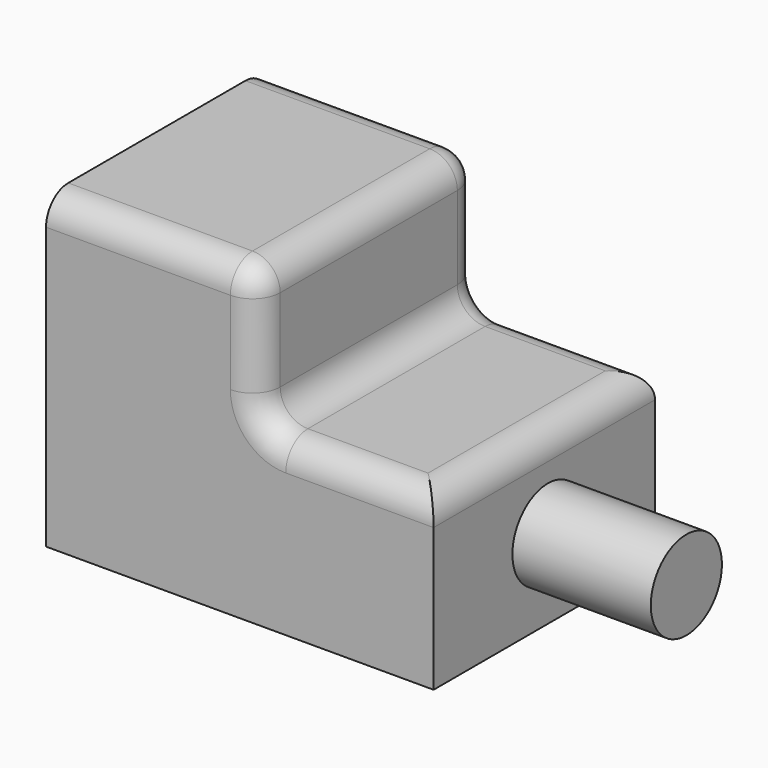
from build123d import *

# Parameters (mm, degrees)
F0_W     = 70
F0_H     = 50
F1_DEPTH = 55.8
F2_R     = 5
F3_R     = 5
F4_W     = 31.709628962
F4_H     = 40
F5_DEPTH = 25
F6_R     = 5
F7_R     = 8.0311344771
F8_DEPTH = 25


with BuildPart() as f1:
    # F0 (on Top) → F1 (new body)
    with BuildSketch(Plane.XY):
        with Locations((-9.0379202738, -0.8199248582)):
            Rectangle(F0_W, F0_H)
    extrude(amount=F1_DEPTH)

    # F2
    f2_edges = [f1.edges().sort_by_distance(p)[0] for p in [
        (-9.03792, -25.819925, 55.8),
    ]]
    fillet(f2_edges, radius=F2_R)

    # F3
    f3_edges = [f1.edges().sort_by_distance(p)[0] for p in [
        (-9.03792, 24.180075, 55.8),
    ]]
    fillet(f3_edges, radius=F3_R)

    # F4 (on face) → F5 (cut)
    with BuildSketch(Plane.XY.offset(55.8)):
        Polygon((30.625000596, 31.9975502789), (-5.7475492358, 31.9975502789), (-5.7475492358, 19.1800751418), (25.9620797262, 19.1800751418), (25.9620797262, -20.8199248582), (-5.7475492358, -20.8199248582), (-5.7475492358, -34.0563766658), (30.625000596, -34.0563766658), align=None)
        with Locations((10.1072652452, -0.8199248582)):
            Rectangle(F4_W, F4_H)
    extrude(amount=-F5_DEPTH, mode=Mode.SUBTRACT)

    # F6
    f6_edges = [f1.edges().sort_by_distance(p)[0] for p in [
        (10.107265, 24.180075, 30.8),
        (25.96208, -0.819925, 30.8),
        (10.107265, -25.819925, 30.8),
        (-5.747549, -0.819925, 30.8),
        (-5.747549, -0.819925, 55.8),
        (-5.747549, 22.715609, 54.335534),
        (-5.747549, -24.355459, 54.335534),
    ]]
    fillet(f6_edges, radius=F6_R)

    # F7 (on face) → F8 (join)
    with BuildSketch(Plane.YZ.offset(25.9620797262)):
        with Locations((0, 14.312678948)):
            Circle(F7_R)
    extrude(amount=F8_DEPTH)


solid = f1.part
